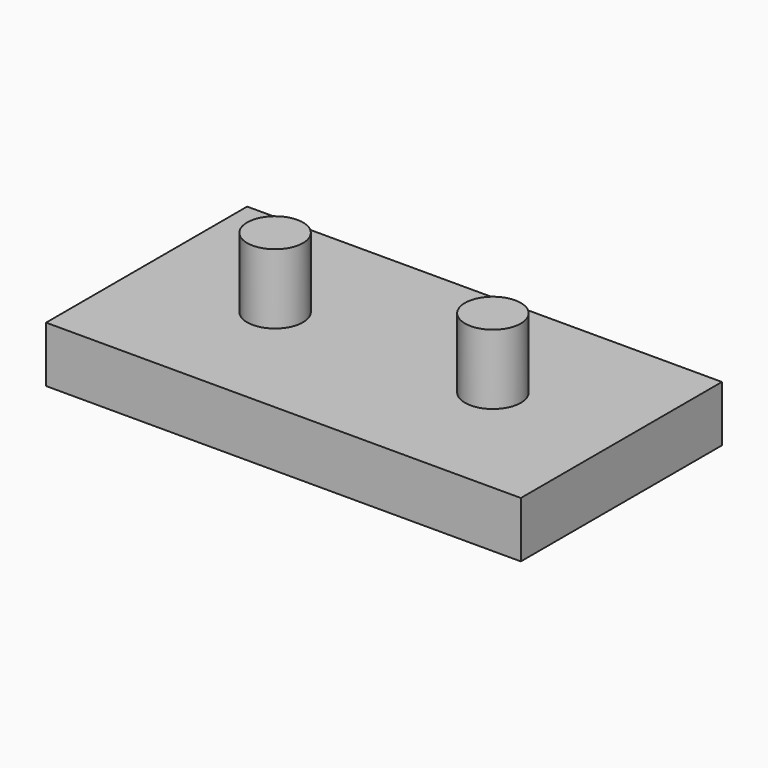
from build123d import *

# Parameters (mm, degrees)
F0_W     = 170
F0_H     = 90
F1_DEPTH = 20
F3_DEPTH = 25


with BuildPart() as f1:
    # F0 (on Top) → F1 (new body)
    with BuildSketch(Plane.XY):
        Rectangle(F0_W, F0_H)
    extrude(amount=F1_DEPTH)

    # F2 (on face) → F3 (join)
    with BuildSketch(Plane.XY.offset(20)):
        with BuildLine():
            Line((-49, 0), (-39, 0))
            Line((-39, 0), (-29, 0))
            ThreePointArc((-29, 0), (-39, 10), (-49, 0))
        make_face()
        with BuildLine():
            Line((-29, 0), (-39, 0))
            Line((-39, 0), (-49, 0))
            ThreePointArc((-49, 0), (-39, -10), (-29, 0))
        make_face()
        with BuildLine():
            ThreePointArc((49, 0), (39, 10), (29, 0))
            Line((29, 0), (39, 0))
            Line((39, 0), (49, 0))
        make_face()
        with BuildLine():
            Line((39, 0), (29, 0))
            ThreePointArc((29, 0), (39, -10), (49, 0))
            Line((49, 0), (39, 0))
        make_face()
    extrude(amount=F3_DEPTH)


solid = f1.part
